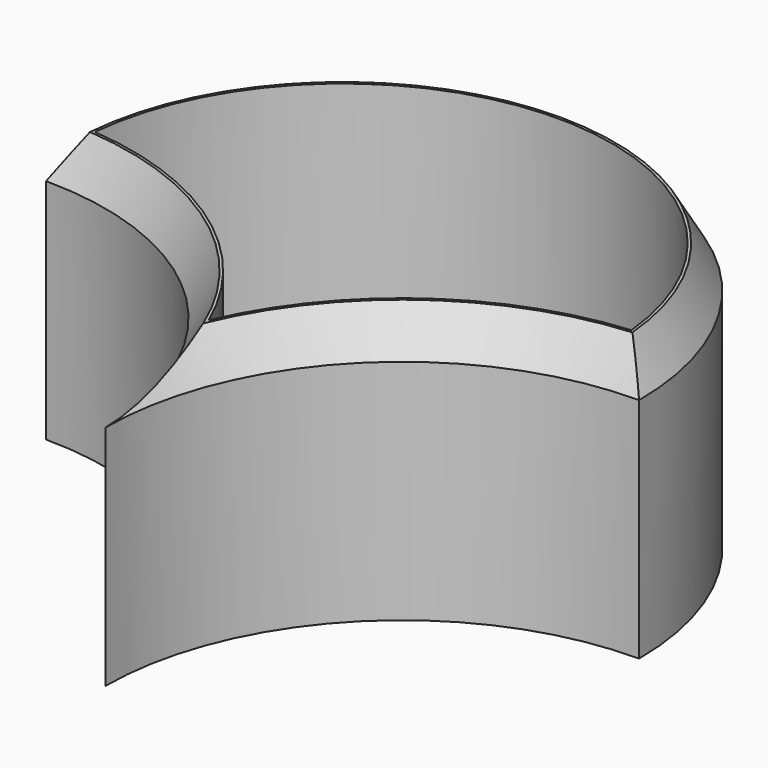
from build123d import *

# Parameters (mm, degrees)
F1_DEPTH    = 25.4
F2_T        = -2.54
F3_T2_ANGLE = 222.0796162883
F3_T4_ANGLE = 132.0289295476
F3_T6_ANGLE = 132.0289295476
F5_DEPTH    = 2.54


# Not quite as in the source:
# - a fillet or chamfer that OpenCascade refuses, or shapes differently, is made with other operations: its cross-section is extruded or revolved along the edge and cut away or added


with BuildPart() as f1:
    # F0 (on Top) → F1 (new body)
    with BuildSketch(Plane.XY):
        with BuildLine():
            ThreePointArc((-27.94, 0), (-8.1834365336, -8.1834365336), (0, -27.94))
            ThreePointArc((0, -27.94), (8.1834365336, -8.1834365336), (27.94, 0))
            ThreePointArc((27.94, 0), (0, 27.94), (-27.94, 0))
        make_face()
    extrude(amount=F1_DEPTH)

    # F2
    f2_openings = [f1.faces().sort_by_distance(p)[0] for p in [
        (0, 7.974025, 25.4),
    ]]
    offset(amount=F2_T, openings=f2_openings)

    # F3: chamfer of 2.286 x 3.9594681461 on 3 edges, made by hand

    # F3_s1 → F3_t2 (revolve, cut)
    with BuildSketch(Plane(origin=(0, 0, 0), x_dir=(0, 0, 1), z_dir=(-0.359016499, -0.9333312132, 0))):
        Polygon((21.4405318539, -27.94), (25.4, -25.654), (25.4, -27.94), align=None)
    revolve(axis=Axis((0, 0, 25.4), (0, 0, 1)), revolution_arc=F3_T2_ANGLE, mode=Mode.SUBTRACT)

    # F3_s3 → F3_t4 (revolve, cut)
    with BuildSketch(Plane(origin=(-33.70000734, -12.9459832215, 0), x_dir=(0, 0, 1), z_dir=(-0.9334899239, -0.3586036279, 0))):
        Polygon((21.4405318539, 11.8776768894), (25.4, 14.1636768894), (25.4, 11.8776768894), align=None)
    revolve(axis=Axis((-27.94, -27.94, 25.4), (0, 0, -1)), revolution_arc=F3_T4_ANGLE, mode=Mode.SUBTRACT)

    # F3_s5 → F3_t6 (revolve, cut)
    with BuildSketch(Plane(origin=(12.9459832215, -33.70000734, 0), x_dir=(0, 0, 1), z_dir=(0.3586036279, -0.9334899239, 0))):
        Polygon((21.4405318539, 11.8776768894), (25.4, 14.1636768894), (25.4, 11.8776768894), align=None)
    revolve(axis=Axis((27.94, -27.94, 25.4), (0, 0, -1)), revolution_arc=F3_T6_ANGLE, mode=Mode.SUBTRACT)

    # F4 (on face) → F5 (cut, through all)
    with BuildSketch(Plane(origin=(0, 0, 0), x_dir=(1, 0, 0), z_dir=(0, 0, -1))):
        with BuildLine():
            ThreePointArc((-20.8487433266, -5.6087433266), (0, -21.59), (20.8487433266, -5.6087433266))
            ThreePointArc((20.8487433266, -5.6087433266), (9.138001762, -0.7355812889), (0, 8.06135568))
            ThreePointArc((0, 8.06135568), (-9.138001762, -0.7355812889), (-20.8487433266, -5.6087433266))
        make_face()
    extrude(amount=-F5_DEPTH, mode=Mode.SUBTRACT)


solid = f1.part
